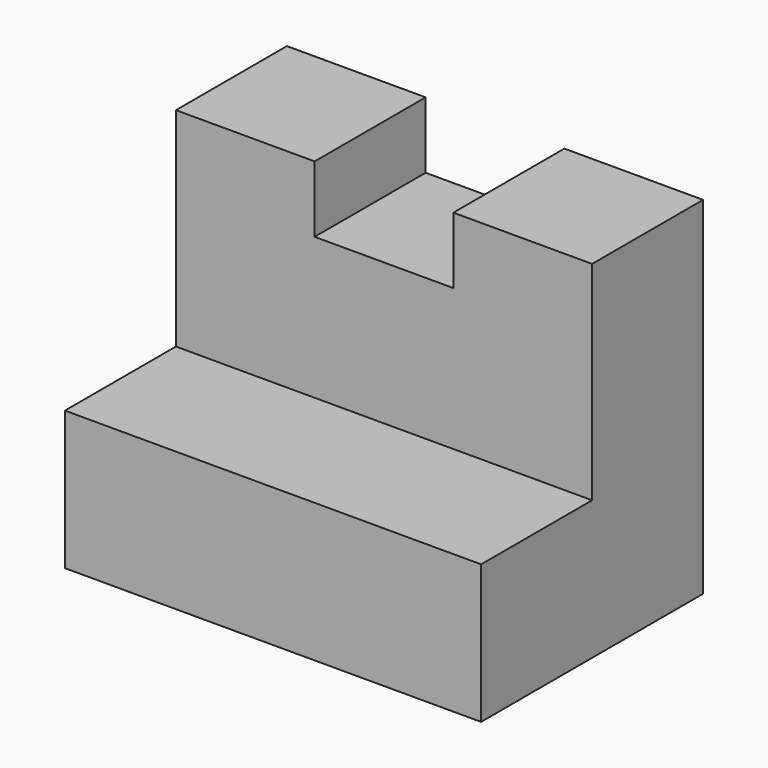
from build123d import *

# Parameters (mm, degrees)
F1_DEPTH = 38.1
F2_W     = 12.7
F2_H     = 12.7
F3_DEPTH = 25.4
F4_W     = 12.7
F4_H     = 6.35
F5_DEPTH = 25.4


# Not quite as in the source:
# - a feature names something its author has since deleted; it is built from what else it names


with BuildPart() as f1:
    # F0 (on Right) → F1 (new body)
    with BuildSketch(Plane.YZ):
        Polygon((-25.4, 0), (0, 0), (0, 31.75), (-12.7, 31.75), (-12.7, 12.7), (-25.4, 12.7), align=None)
    extrude(amount=F1_DEPTH)

    # F2 (on Top) → F3 (join)
    with BuildSketch(Plane.XY):
        with Locations((19.05, -6.35)):
            Rectangle(F2_W, F2_H)
    extrude(amount=F3_DEPTH)

    # F4 (on Front) → F5 (cut)
    with BuildSketch(Plane.XZ):
        with Locations((19.05, 28.8461486514)):
            Rectangle(F4_W, F4_H)
    extrude(amount=F5_DEPTH, mode=Mode.SUBTRACT)


solid = f1.part
